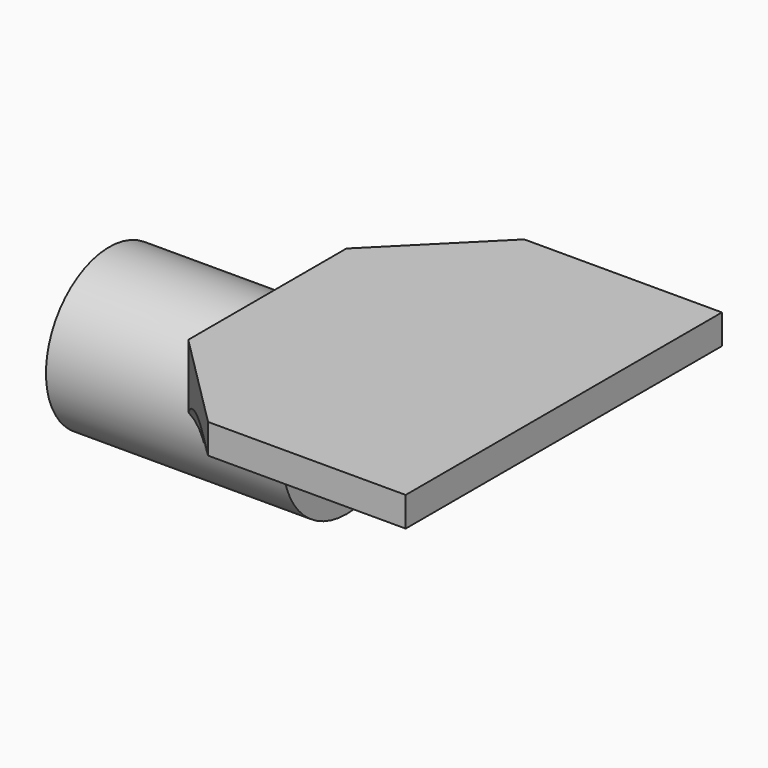
from build123d import *

# Parameters (mm, degrees)
F0_R        = 4
F0_R_2      = 1.5
F1_DEPTH    = 10
F2_R        = 4
F3_DEPTH    = 2
F4_W        = 15
F4_H        = 1.5
F5_DEPTH    = 10
F6_T1_DEPTH = 4
F7_SIZE     = 5


# Not quite as in the source:
# - a fillet or chamfer that OpenCascade refuses, or shapes differently, is made with other operations: its cross-section is extruded or revolved along the edge and cut away or added


with BuildPart() as f1:
    # F0 (on Right) → F1 (new body)
    with BuildSketch(Plane.YZ):
        Circle(F0_R)
        Circle(F0_R_2, mode=Mode.SUBTRACT)
    extrude(amount=F1_DEPTH)

    # F2 (on face) → F3 (join)
    with BuildSketch(Plane.YZ.offset(10)):
        Circle(F2_R)
    extrude(amount=F3_DEPTH)

    # F4 (on Front) → F5 (join, symmetric)
    with BuildSketch(Plane.XZ):
        with Locations((15.5, 3.75)):
            Rectangle(F4_W, F4_H)
    extrude(amount=F5_DEPTH, both=True)

    # F6: fillet of radius 5 on 2 edges, made by hand

    # F6_s2 → F6_t1 (join)
    with BuildSketch(Plane.YZ.offset(8)):
        with BuildLine():
            ThreePointArc((-3.8999841722, -0.8888888889), (-5.6569165651, 1.9086797999), (-8.7749643874, 3))
            Line((-8.7749643874, 3), (-2.6457513111, 3))
            ThreePointArc((-2.6457513111, 3), (-3.8069052328, 1.2277917365), (-3.8999841722, -0.8888888889))
        make_face()
        with BuildLine():
            ThreePointArc((3.8999841722, -0.8888888889), (5.6569165651, 1.9086797999), (8.7749643874, 3))
            Line((8.7749643874, 3), (2.6457513111, 3))
            ThreePointArc((2.6457513111, 3), (3.8069052328, 1.2277917365), (3.8999841722, -0.8888888889))
        make_face()
    extrude(amount=F6_T1_DEPTH)

    # F7
    f7_edges = [f1.edges().sort_by_distance(p)[0] for p in [
        (8, 10, 3.75),
        (8, -10, 3.75),
    ]]
    chamfer(f7_edges, length=F7_SIZE)


solid = f1.part
